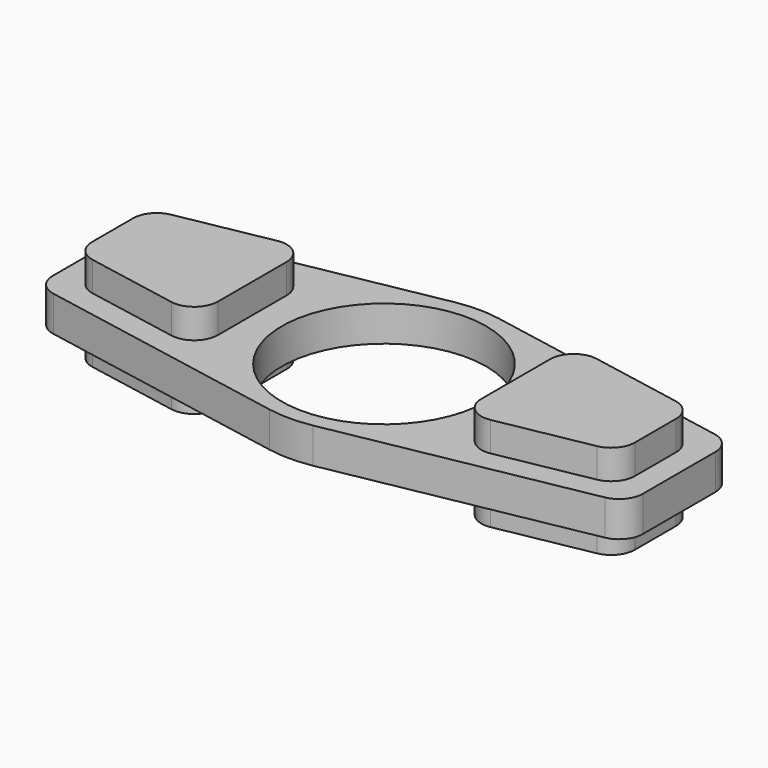
from build123d import *

# Parameters (mm, degrees)
F0_R             = 11
F1_DEPTH         = 1.905
F3_R             = 2.54
F4_DEPTH         = 3.175
F4_COPIES2_COUNT = 2
F5_R             = 2.54


# Not quite as in the source:
# - a pattern or mirror of a feature is missing from the dataset's text; its kind, count and spacing are read off the source's solid


with BuildPart() as f1:
    # F0 (on Top) → F1 (new body, symmetric)
    with BuildSketch(Plane.XY):
        with BuildLine():
            Line((-31.75, -6.9869237544), (-2.3327823548, -12.4839147099))
            ThreePointArc((-2.3327823548, -12.4839147099), (0, -12.7), (2.3327823548, -12.4839147099))
            Line((2.3327823548, -12.4839147099), (31.75, -6.9869237544))
            Line((31.75, -6.9869237544), (31.75, 6.9869237544))
            Line((31.75, 6.9869237544), (2.3327823548, 12.4839147099))
            ThreePointArc((2.3327823548, 12.4839147099), (0, 12.7), (-2.3327823548, 12.4839147099))
            Line((-2.3327823548, 12.4839147099), (-31.75, 6.9869237544))
            Line((-31.75, 6.9869237544), (-31.75, -6.9869237544))
        make_face()
        Circle(F0_R, mode=Mode.SUBTRACT)
    extrude(amount=F1_DEPTH, both=True)

    # F3
    f3_edges = [f1.edges().sort_by_distance(p)[0] for p in [
        (-31.75, 6.986924, 0),
        (-31.75, -6.986924, 0),
        (31.75, -6.986924, 0),
        (31.75, 6.986924, 0),
    ]]
    fillet(f3_edges, radius=F3_R)

    # F2 (on face) → F4 (join)
    with BuildSketch(Plane.XY.offset(1.905)):
        Polygon((-29.21, 4.8775907903), (-29.21, -4.8775907903), (-14.175, -7.6870767183), (-14.175, 7.6870767183), align=None)
    f4 = extrude(amount=F4_DEPTH)

    # F4_copies: F4 across plane
    add(f4.mirror(Plane(origin=(0, 0, 0), x_dir=(0, 0, 1), z_dir=(1, 0, 0))))

    # F4_copies1: F4 across plane
    add(f4.mirror(Plane(origin=(0, 0, 0), x_dir=(-1, 0, 0), z_dir=(0, 0, -1))))

    # F4_copies2: F4 ×2 about axis
    f4_copies2_axis = Axis((0, 0, 0), (0, 1, 0))
    for i in range(1, F4_COPIES2_COUNT):
        add(f4.rotate(f4_copies2_axis, i * 360 / F4_COPIES2_COUNT))

    # F5
    f5_edges = [f1.edges().sort_by_distance(p)[0] for p in [
        (-29.21, -4.877591, 3.4925),
        (-14.175, -7.687077, 3.4925),
        (-14.175, 7.687077, 3.4925),
        (-29.21, 4.877591, 3.4925),
        (-14.175, -7.687077, -3.4925),
        (-14.175, 7.687077, -3.4925),
        (-29.21, -4.877591, -3.4925),
        (-29.21, 4.877591, -3.4925),
        (29.21, -4.877591, -3.4925),
        (14.175, -7.687077, -3.4925),
        (29.21, 4.877591, -3.4925),
        (14.175, 7.687077, -3.4925),
        (29.21, -4.877591, 3.4925),
        (14.175, -7.687077, 3.4925),
        (29.21, 4.877591, 3.4925),
        (14.175, 7.687077, 3.4925),
    ]]
    fillet(f5_edges, radius=F5_R)


solid = f1.part
